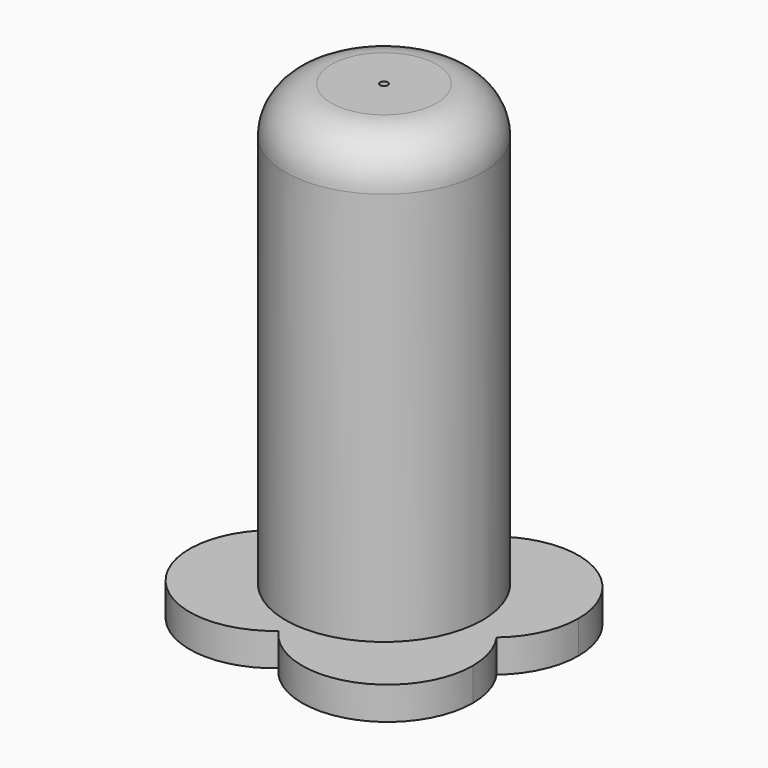
from build123d import *

# Parameters (mm, degrees)
F1_DEPTH  = 60
F2_DEPTH  = 5
F3_R      = 15
F4_DEPTH  = 8
F5_R      = 1.5
F6_DEPTH  = 68.001
F7_R      = 15
F8_DEPTH  = 4
F9_R      = 0.6
F11_DEPTH = 72.001


# Not quite as in the source:
# - a fillet or chamfer that OpenCascade refuses, or shapes differently, is made with other operations: its cross-section is extruded or revolved along the edge and cut away or added


with BuildPart() as f1:
    # F0 (on Top) → F1 (new body)
    with BuildSketch(Plane.XY):
        with BuildLine():
            ThreePointArc((4.344342247, 12.2526197379), (9.8886206176, 8.4389088324), (12.7832510794, 2.3639991203))
            ThreePointArc((12.7832510794, 2.3639991203), (13.8829504808, 1.9165651298), (14.9372441283, 1.3706705849))
            ThreePointArc((14.9372441283, 1.3706705849), (11.4099468664, 9.7372024989), (3.7020104756, 14.5359938923))
            ThreePointArc((3.7020104756, 14.5359938923), (4.0753636897, 13.4089875362), (4.344342247, 12.2526197379))
        make_face()
        with BuildLine():
            ThreePointArc((12.7832510794, 2.3639991203), (12.9456993637, 1.1869574482), (13, 0))
            ThreePointArc((13, 0), (12.6914373848, -2.8155669247), (11.7803973681, -5.4974755888))
            ThreePointArc((11.7803973681, -5.4974755888), (12.9572055714, -5.3404456491), (14.1147802532, -5.0767094072))
            ThreePointArc((14.1147802532, -5.0767094072), (14.7770379948, -2.5766544396), (15, 0))
            ThreePointArc((15, 0), (14.9843028187, 0.6860532326), (14.9372441283, 1.3706705849))
            ThreePointArc((14.9372441283, 1.3706705849), (13.8829504808, 1.9165651298), (12.7832510794, 2.3639991203))
        make_face()
        with BuildLine():
            ThreePointArc((14.1147802532, -5.0767094072), (12.9572055714, -5.3404456491), (11.7803973681, -5.4974755888))
            ThreePointArc((11.7803973681, -5.4974755888), (7.453385593, -10.6511522007), (1.1292451674, -12.9508611819))
            ThreePointArc((1.1292451674, -12.9508611819), (0.5785791746, -14.0026705342), (-0.0657478246, -14.9998559068))
            ThreePointArc((-0.0657478246, -14.9998559068), (8.6000602997, -12.2897910008), (14.1147802532, -5.0767094072))
        make_face()
        with BuildLine():
            ThreePointArc((-0.0657478246, -14.9998559068), (0.5785791746, -14.0026705342), (1.1292451674, -12.9508611819))
            ThreePointArc((1.1292451674, -12.9508611819), (-1.6450220625, -12.8954993084), (-4.344342247, -12.2526197379))
            ThreePointArc((-4.344342247, -12.2526197379), (-4.0753636897, -13.4089875362), (-3.7020104756, -14.5359938923))
            ThreePointArc((-3.7020104756, -14.5359938923), (-1.8981023799, -14.879422279), (-0.0657478246, -14.9998559068))
        make_face()
        with BuildLine():
            ThreePointArc((-3.7020104756, -14.5359938923), (-4.0753636897, -13.4089875362), (-4.344342247, -12.2526197379))
            ThreePointArc((-4.344342247, -12.2526197379), (-9.8886206176, -8.4389088324), (-12.7832510794, -2.3639991203))
            ThreePointArc((-12.7832510794, -2.3639991203), (-13.8829504808, -1.9165651298), (-14.9372441283, -1.3706705849))
            ThreePointArc((-14.9372441283, -1.3706705849), (-11.4099468664, -9.7372024989), (-3.7020104756, -14.5359938923))
        make_face()
        with BuildLine():
            ThreePointArc((-12.7832510794, -2.3639991203), (-12.8954993084, 1.6450220625), (-11.7803973681, 5.4974755888))
            ThreePointArc((-11.7803973681, 5.4974755888), (-12.9572055714, 5.3404456491), (-14.1147802532, 5.0767094072))
            ThreePointArc((-14.1147802532, 5.0767094072), (-14.879422279, 1.8981023799), (-14.9372441283, -1.3706705849))
            ThreePointArc((-14.9372441283, -1.3706705849), (-13.8829504808, -1.9165651298), (-12.7832510794, -2.3639991203))
        make_face()
        with BuildLine():
            ThreePointArc((-11.7803973681, 5.4974755888), (-7.453385593, 10.6511522007), (-1.1292451674, 12.9508611819))
            ThreePointArc((-1.1292451674, 12.9508611819), (-0.5785791746, 14.0026705342), (0.0657478246, 14.9998559068))
            ThreePointArc((0.0657478246, 14.9998559068), (-8.6000602997, 12.2897910008), (-14.1147802532, 5.0767094072))
            ThreePointArc((-14.1147802532, 5.0767094072), (-12.9572055714, 5.3404456491), (-11.7803973681, 5.4974755888))
        make_face()
        with BuildLine():
            ThreePointArc((-1.1292451674, 12.9508611819), (1.6450220625, 12.8954993084), (4.344342247, 12.2526197379))
            ThreePointArc((4.344342247, 12.2526197379), (4.0753636897, 13.4089875362), (3.7020104756, 14.5359938923))
            ThreePointArc((3.7020104756, 14.5359938923), (1.8981023799, 14.879422279), (0.0657478246, 14.9998559068))
            ThreePointArc((0.0657478246, 14.9998559068), (-0.5785791746, 14.0026705342), (-1.1292451674, 12.9508611819))
        make_face()
    extrude(amount=F1_DEPTH)

    # F0 (on Top) → F2 (join)
    with BuildSketch(Plane.XY):
        with BuildLine():
            ThreePointArc((3.7020104756, 14.5359938923), (11.4099468664, 9.7372024989), (14.9372441283, 1.3706705849))
            ThreePointArc((14.9372441283, 1.3706705849), (17.2222714986, -0.3046475231), (19.0900610331, -2.4352350245))
            ThreePointArc((19.0900610331, -2.4352350245), (22.4559354435, 2.0084712145), (23.6511522007, 7.453385593))
            ThreePointArc((23.6511522007, 7.453385593), (16.0960665792, 19.2581688359), (2.2122433682, 17.3420062106))
            ThreePointArc((2.2122433682, 17.3420062106), (3.0431666419, 15.9846802304), (3.7020104756, 14.5359938923))
        make_face()
        with BuildLine():
            ThreePointArc((19.0900610331, -2.4352350245), (17.2222714986, -0.3046475231), (14.9372441283, 1.3706705849))
            ThreePointArc((14.9372441283, 1.3706705849), (14.9843028187, 0.6860532326), (15, 0))
            ThreePointArc((15, 0), (14.7770379948, -2.5766544396), (14.1147802532, -5.0767094072))
            ThreePointArc((14.1147802532, -5.0767094072), (16.7472118135, -4.0286898812), (19.0900610331, -2.4352350245))
        make_face()
        with BuildLine():
            ThreePointArc((19.0900610331, -2.4352350245), (16.7472118135, -4.0286898812), (14.1147802532, -5.0767094072))
            ThreePointArc((14.1147802532, -5.0767094072), (8.6000602997, -12.2897910008), (-0.0657478246, -14.9998559068))
            ThreePointArc((-0.0657478246, -14.9998559068), (-1.0671791062, -16.2367482592), (-2.2122433682, -17.3420062106))
            ThreePointArc((-2.2122433682, -17.3420062106), (12.346275042, -22.2875112657), (21.4389088324, -9.8886206176))
            ThreePointArc((21.4389088324, -9.8886206176), (20.8377994805, -5.981254408), (19.0900610331, -2.4352350245))
        make_face()
        with BuildLine():
            ThreePointArc((0.0657478246, 14.9998559068), (1.8981023799, 14.879422279), (3.7020104756, 14.5359938923))
            ThreePointArc((3.7020104756, 14.5359938923), (3.0431666419, 15.9846802304), (2.2122433682, 17.3420062106))
            ThreePointArc((2.2122433682, 17.3420062106), (1.0671791062, 16.2367482592), (0.0657478246, 14.9998559068))
        make_face()
        with BuildLine():
            ThreePointArc((-2.2122433682, -17.3420062106), (-1.0671791062, -16.2367482592), (-0.0657478246, -14.9998559068))
            ThreePointArc((-0.0657478246, -14.9998559068), (-1.8981023799, -14.879422279), (-3.7020104756, -14.5359938923))
            ThreePointArc((-3.7020104756, -14.5359938923), (-3.0431666419, -15.9846802304), (-2.2122433682, -17.3420062106))
        make_face()
        with BuildLine():
            ThreePointArc((-14.1147802532, 5.0767094072), (-8.6000602997, 12.2897910008), (0.0657478246, 14.9998559068))
            ThreePointArc((0.0657478246, 14.9998559068), (1.0671791062, 16.2367482592), (2.2122433682, 17.3420062106))
            ThreePointArc((2.2122433682, 17.3420062106), (-15.8922944255, 20.5397728182), (-19.0900610331, 2.4352350245))
            ThreePointArc((-19.0900610331, 2.4352350245), (-16.7472118135, 4.0286898812), (-14.1147802532, 5.0767094072))
        make_face()
        with BuildLine():
            ThreePointArc((-2.2122433682, -17.3420062106), (-3.0431666419, -15.9846802304), (-3.7020104756, -14.5359938923))
            ThreePointArc((-3.7020104756, -14.5359938923), (-11.4099468664, -9.7372024989), (-14.9372441283, -1.3706705849))
            ThreePointArc((-14.9372441283, -1.3706705849), (-17.2222714986, 0.3046475231), (-19.0900610331, 2.4352350245))
            ThreePointArc((-19.0900610331, 2.4352350245), (-20.5397728182, -15.8922944255), (-2.2122433682, -17.3420062106))
        make_face()
        with BuildLine():
            ThreePointArc((-14.9372441283, -1.3706705849), (-14.879422279, 1.8981023799), (-14.1147802532, 5.0767094072))
            ThreePointArc((-14.1147802532, 5.0767094072), (-16.7472118135, 4.0286898812), (-19.0900610331, 2.4352350245))
            ThreePointArc((-19.0900610331, 2.4352350245), (-17.2222714986, 0.3046475231), (-14.9372441283, -1.3706705849))
        make_face()
    extrude(amount=F2_DEPTH)

    # F3 (on face) → F4 (join)
    with BuildSketch(Plane.XY.offset(60)):
        Circle(F3_R)
    extrude(amount=F4_DEPTH)

    # F5 (on face) → F6 (cut, through all)
    with BuildSketch(Plane.XY.offset(68)):
        Circle(F5_R)
    extrude(amount=-F6_DEPTH, mode=Mode.SUBTRACT)

    # F7 (on face) → F8 (join)
    with BuildSketch(Plane.XY.offset(68)):
        Circle(F7_R)
    extrude(amount=F8_DEPTH)

    # F10: fillet of radius 7 on 1 edges, made by hand

    # F10_s1 → F10_t2 (revolve, cut)
    with BuildSketch(Plane.XZ):
        with BuildLine():
            ThreePointArc((15, 65), (12.9497474683, 69.9497474683), (8, 72))
            Line((8, 72), (15, 72))
            Line((15, 72), (15, 65))
        make_face()
    revolve(axis=Axis((0, 0, 72), (0, 0, 1)), mode=Mode.SUBTRACT)

    # F9 (on face) → F11 (cut, through all)
    with BuildSketch(Plane.XY.offset(72)):
        Circle(F9_R)
    extrude(amount=-F11_DEPTH, mode=Mode.SUBTRACT)


solid = f1.part
